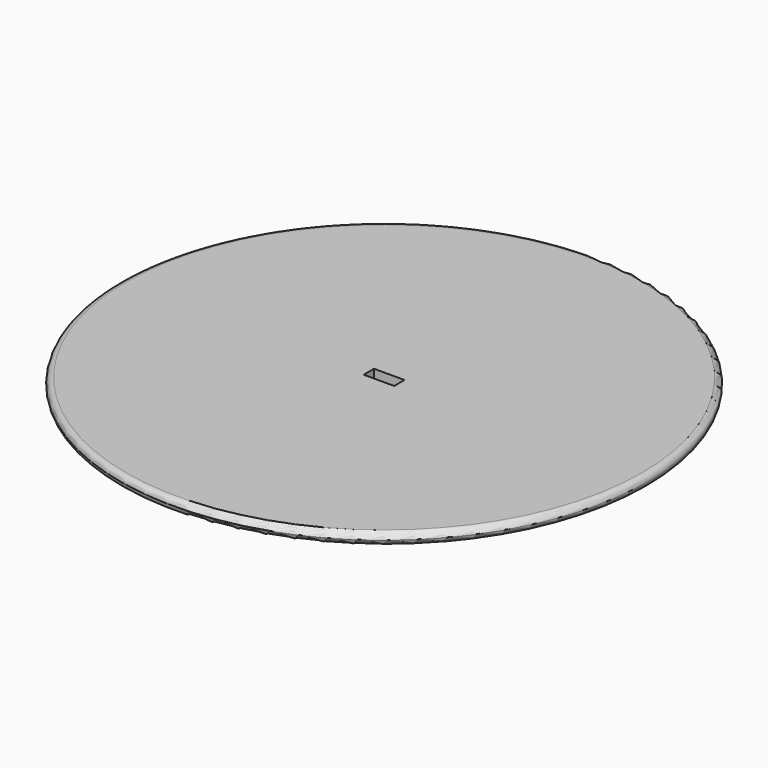
from build123d import *

# Parameters (mm, degrees)
F0_R     = 45
F0_W     = 5.2
F0_H     = 2.2
F1_DEPTH = 2
F2_R     = 1
F3_R     = 0.99999
F4_R     = 0.5


# Not quite as in the source:
# - a fillet or chamfer is up to 0.001 mm smaller than in the source, because OpenCascade refuses the exact size


with BuildPart() as f1:
    # F0 (on Top) → F1 (new body)
    with BuildSketch(Plane.XY):
        Circle(F0_R)
        Rectangle(F0_W, F0_H, mode=Mode.SUBTRACT)
    extrude(amount=F1_DEPTH)

    # F2
    f2_edges = [f1.edges().sort_by_distance(p)[0] for p in [
        (-45, 0, 2),
    ]]
    fillet(f2_edges, radius=F2_R)

    # F3 (radius 1 in the source; OpenCascade refuses exactly that, so slightly less here)
    f3_edges = [f1.edges().sort_by_distance(p)[0] for p in [
        (-45, 0, 0),
    ]]
    fillet(f3_edges, radius=F3_R)

    # F4
    f4_edges = [f1.edges().sort_by_distance(p)[0] for p in [
        (-2.6, 0, 0),
        (0, -1.1, 0),
        (2.6, 0, 0),
        (0, 1.1, 0),
    ]]
    fillet(f4_edges, radius=F4_R)


solid = f1.part
